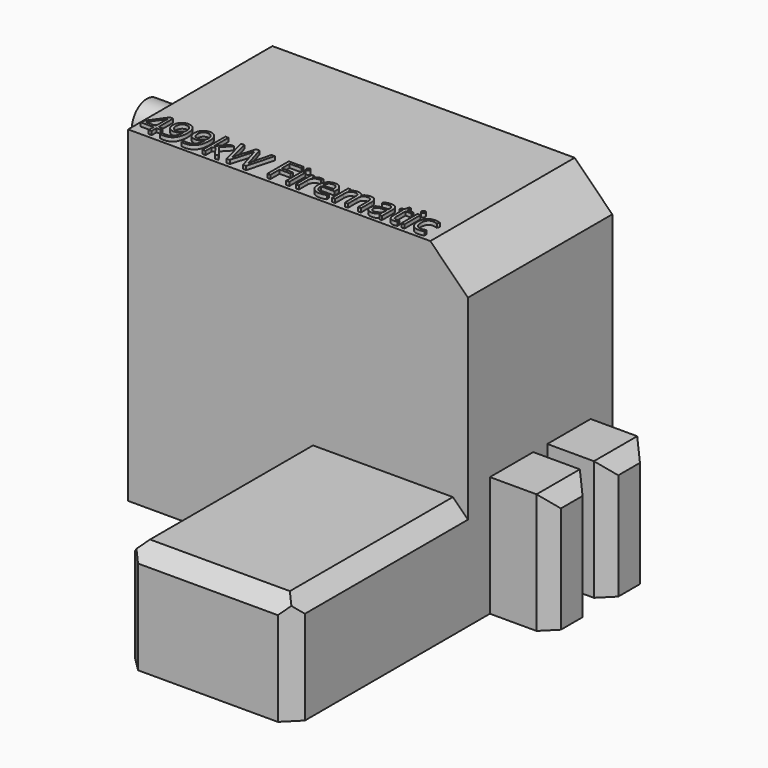
from build123d import *

# Parameters (mm, degrees)
F0_W         = 2260
F0_H         = 1200
F1_DEPTH     = 2175
F2_TEXT_SIZE = 250
F3_DEPTH     = 25
F4_W         = 1130
F4_H         = 725
F5_DEPTH     = 1455
F6_C1_SIZE   = 100
F6_C2_SIZE   = 100
F6_C3_SIZE   = 100
F6_C4_SIZE   = 100
F6_C5_SIZE   = 100
F8_W         = 360
F8_H         = 800
F9_DEPTH     = 400
F10_SIZE     = 90
F11_W        = 360
F11_H        = 800
F12_DEPTH    = 400
F13_SIZE     = 90
F14_R        = 125
F15_DEPTH    = 355
F16_SIZE     = 250


# Not quite as in the source:
# - two fillets or chamfers of one size are made in one step
# - Text() gives the source's letters only with a copy of the font that has no kerning and outlines rounded to 1/6400 em; it was checked with that copy


with BuildPart() as f1:
    # F0 (on Top) → F1 (new body)
    with BuildSketch(Plane.XY):
        with Locations((1130, 600)):
            Rectangle(F0_W, F0_H)
    extrude(amount=F1_DEPTH)

    # F2 (on face) → F3 (join)
    with BuildSketch(Plane.XY.offset(2175)):
        with Locations((25, 25)):
            Text('499kW Firematic', F2_TEXT_SIZE, font='Open Sans', text_align=(TextAlign.LEFT, TextAlign.BOTTOM))
    extrude(amount=F3_DEPTH)

    # F4 (on face) → F5 (join)
    with BuildSketch(Plane.XZ):
        with Locations((1695, 362.5)):
            Rectangle(F4_W, F4_H)
    extrude(amount=F5_DEPTH)

    # F6: chamfer of 100 on 5 edges, made by hand

    # F6_c1
    f6_c1_edges = [f1.edges().sort_by_distance(p)[0] for p in [
        (2260, -1455, 362.5),
    ]]
    chamfer(f6_c1_edges, length=F6_C1_SIZE)

    # F6_c2
    f6_c2_edges = [f1.edges().sort_by_distance(p)[0] for p in [
        (2260, -677.5, 725),
    ]]
    chamfer(f6_c2_edges, length=F6_C2_SIZE)

    # F6_c3
    f6_c3_edges = [f1.edges().sort_by_distance(p)[0] for p in [
        (1130, -727.5, 725),
    ]]
    chamfer(f6_c3_edges, length=F6_C3_SIZE)

    # F6_c4
    f6_c4_edges = [f1.edges().sort_by_distance(p)[0] for p in [
        (1695, -1455, 725),
    ]]
    chamfer(f6_c4_edges, length=F6_C4_SIZE)

    # F6_c5
    f6_c5_edges = [f1.edges().sort_by_distance(p)[0] for p in [
        (1130, -1455, 312.5),
    ]]
    chamfer(f6_c5_edges, length=F6_C5_SIZE)

    # F8 (on face) → F9 (join)
    with BuildSketch(Plane.YZ.offset(2260)):
        with Locations((363, 400)):
            Rectangle(F8_W, F8_H)
    extrude(amount=F9_DEPTH)

    # F10
    f10_edges = [f1.edges().sort_by_distance(p)[0] for p in [
        (2660, 183, 400),
        (2660, 363, 800),
        (2660, 543, 400),
    ]]
    chamfer(f10_edges, length=F10_SIZE)

    # F11 (on face) → F12 (join, through all)
    with BuildSketch(Plane.YZ.offset(2260)):
        with Locations((840, 400)):
            Rectangle(F11_W, F11_H)
    extrude(amount=F12_DEPTH)

    # F13
    f13_edges = [f1.edges().sort_by_distance(p)[0] for p in [
        (2660, 1020, 400),
        (2660, 840, 800),
        (2660, 660, 400),
    ]]
    chamfer(f13_edges, length=F13_SIZE)

    # F14 (on face) → F15 (join)
    with BuildSketch(Plane(origin=(0, 0, 0), x_dir=(0, -1, 0), z_dir=(-1, 0, 0))):
        with Locations((-600, 1870)):
            Circle(F14_R)
    extrude(amount=F15_DEPTH)

    # F16
    f16_edges = [f1.edges().sort_by_distance(p)[0] for p in [
        (2260, 600, 2175),
    ]]
    chamfer(f16_edges, length=F16_SIZE)


solid = f1.part
